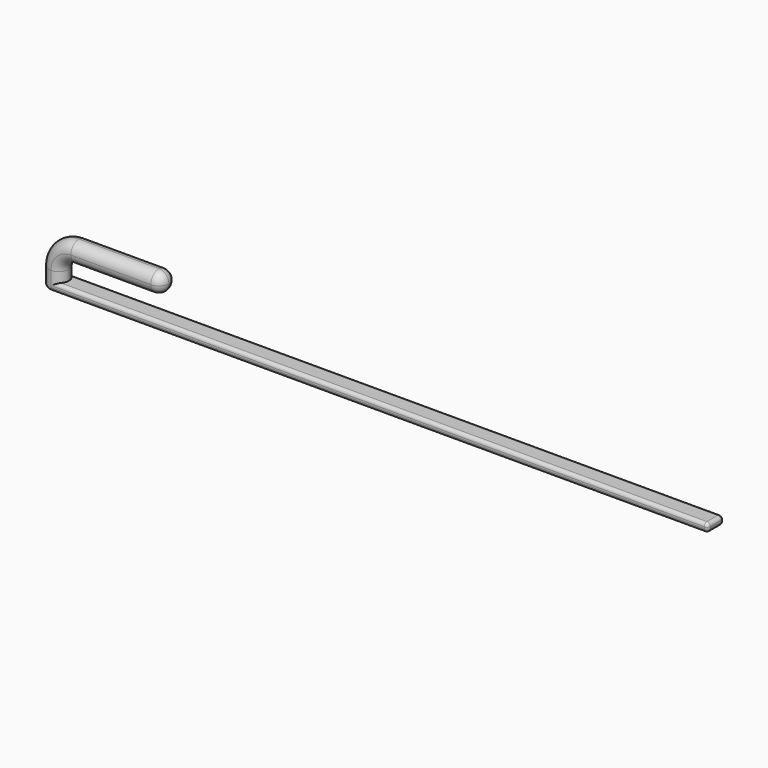
from build123d import *

# Parameters (mm, degrees)
F1_DEPTH = 7.62
F2_R     = 3.80999
F3_R     = 3.80999
F4_R     = 1.27
F5_R     = 1.27


# Not quite as in the source:
# - a fillet or chamfer is up to 0.001 mm smaller than in the source, because OpenCascade refuses the exact size


with BuildPart() as f1:
    # F0 (on Front) → F1 (new body)
    with BuildSketch(Plane.XZ):
        with BuildLine():
            Line((134.7724028379, 37.2032584392), (-111.6075971621, 37.2032584392))
            Line((-111.6075971621, 37.2032584392), (-111.6075971621, 41.0132584392))
            ThreePointArc((-111.6075971621, 41.0132584392), (-110.4916739984, 43.7073352756), (-107.7975971621, 44.8232584392))
            Line((-107.7975971621, 44.8232584392), (-73.5075971621, 44.8232584392))
            Line((-73.5075971621, 44.8232584392), (-73.5075971621, 52.4432584392))
            Line((-73.5075971621, 52.4432584392), (-107.7975971621, 52.4432584392))
            ThreePointArc((-107.7975971621, 52.4432584392), (-115.8798276711, 49.0954889482), (-119.2275971621, 41.0132584392))
            Line((-119.2275971621, 41.0132584392), (-119.2275971621, 37.2032584392))
            Line((-119.2275971621, 37.2032584392), (-119.2275971621, 34.0282584392))
            Line((-119.2275971621, 34.0282584392), (134.7724028379, 34.0282584392))
            Line((134.7724028379, 34.0282584392), (134.7724028379, 37.2032584392))
        make_face()
    extrude(amount=F1_DEPTH)

    # F2 (radius 3.81 in the source; OpenCascade refuses exactly that, so slightly less here)
    f2_edges = [f1.edges().sort_by_distance(p)[0] for p in [
        (-90.652597, -7.62, 52.443258),
        (-90.652597, -7.62, 44.823258),
        (-90.652597, 0, 44.823258),
        (-90.652597, 0, 52.443258),
    ]]
    fillet(f2_edges, radius=F2_R)

    # F3 (radius 3.81 in the source; OpenCascade refuses exactly that, so slightly less here)
    f3_edges = [f1.edges().sort_by_distance(p)[0] for p in [
        (-73.507597, -3.81, 52.443258),
        (-73.507597, -1.11592, 51.327338),
        (-73.507597, 0, 48.633258),
        (-73.507597, -1.11592, 45.939179),
        (-73.507597, -3.81, 44.823258),
        (-73.507597, -6.50408, 45.939179),
        (-73.507597, -6.50408, 51.327338),
        (-73.507597, -7.62, 48.633258),
    ]]
    fillet(f3_edges, radius=F3_R)

    # F4
    f4_edges = [f1.edges().sort_by_distance(p)[0] for p in [
        (11.582403, -7.62, 37.203258),
        (9.677398, -7.62, 34.028258),
        (11.582403, 0, 37.203258),
        (9.677398, 0, 34.028258),
    ]]
    fillet(f4_edges, radius=F4_R)

    # F5
    f5_edges = [f1.edges().sort_by_distance(p)[0] for p in [
        (134.772403, -7.248026, 36.831284),
        (134.772403, -7.62, 35.615758),
        (134.772403, -7.248026, 34.400233),
        (134.772403, -3.81, 34.028258),
        (134.772403, -0.371974, 34.400233),
        (134.772403, 0, 35.615758),
        (134.772403, -3.81, 37.203258),
        (134.772403, -0.371974, 36.831284),
    ]]
    fillet(f5_edges, radius=F5_R)


solid = f1.part
